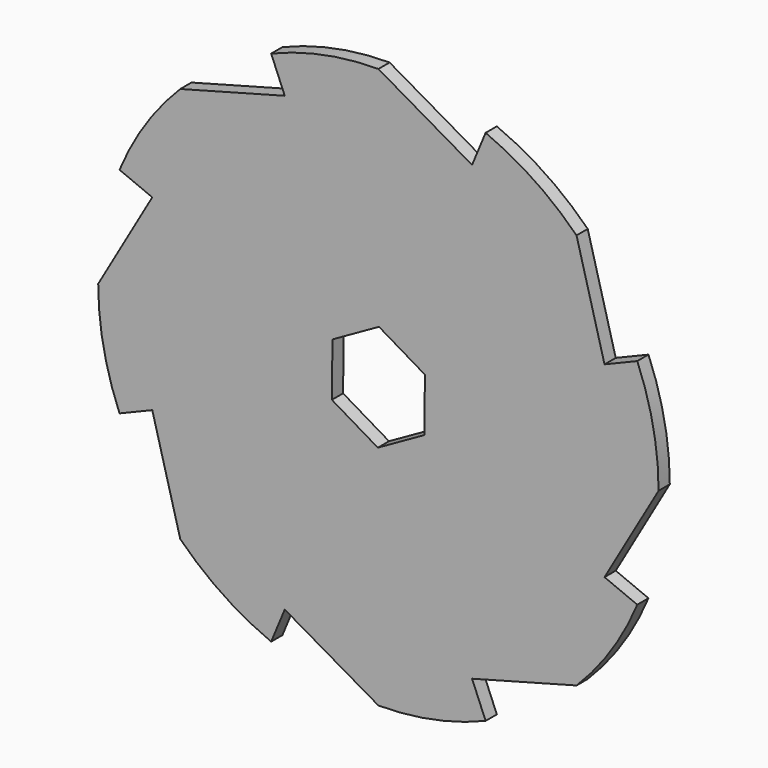
from build123d import *

# Parameters (mm, degrees)
F0_R            = 63.5
F1_DEPTH        = 3.175
F3_DEPTH        = 3.175
F3_COPIES_COUNT = 8
F5_DEPTH        = 3.175


# Not quite as in the source:
# - a pattern or mirror of a feature is missing from the dataset's text; its kind, count and spacing are read off the source's solid


with BuildPart() as f1:
    # F0 (on Front) → F1 (new body)
    with BuildSketch(Plane.XZ):
        Circle(F0_R)
    extrude(amount=F1_DEPTH)

    # F2 (on face) → F3 (cut)
    with BuildSketch(Plane.XZ.offset(3.175)):
        with BuildLine():
            Line((0, 63.5), (21.2263563726, 51.2449574344))
            Line((21.2263563726, 51.2449574344), (24.3003979552, 58.6663503145))
            ThreePointArc((24.3003979552, 58.6663503145), (12.388235448, 62.2798653056), (0, 63.5))
        make_face()
    f3 = extrude(amount=-F3_DEPTH, mode=Mode.SUBTRACT)

    # F3_copies: F3 ×8 about axis
    f3_copies_axis = Axis((0, 0, 0), (0, 1, 0))
    for i in range(1, F3_COPIES_COUNT):
        add(f3.rotate(f3_copies_axis, i * 360 / F3_COPIES_COUNT), mode=Mode.SUBTRACT)

    # F4 (on Front) → F5 (cut)
    with BuildSketch(Plane.XZ):
        Polygon((0.1275317148, 12.0983748909), (-10.4137341426, 6.1596331502), (-10.5412658574, -5.9387417407), (-0.1275317148, -12.0983748909), (10.4137341426, -6.1596331502), (10.5412658574, 5.9387417407), align=None)
    extrude(amount=F5_DEPTH, mode=Mode.SUBTRACT)


solid = f1.part
